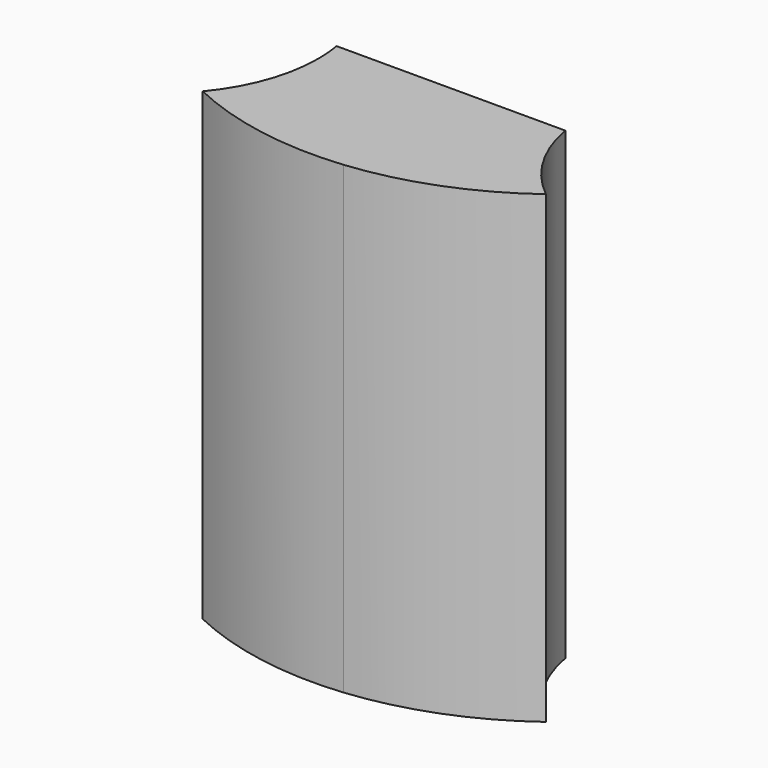
from build123d import *

# Parameters (mm, degrees)
F1_DEPTH = 76.2


with BuildPart() as f1:
    # F0 (on Top) → F1 (new body)
    with BuildSketch(Plane.XY):
        with BuildLine():
            ThreePointArc((5.0166433221, -50.5516892871), (18.3621332827, -47.3653044043), (30.3681236725, -40.7236671312))
            ThreePointArc((30.3681236725, -40.7236671312), (24.4383893444, -33.8843769742), (21.2835539426, -25.4))
            Line((21.2835539426, -25.4), (-16.2238025261, -25.4))
            ThreePointArc((-16.2238025261, -25.4), (-15.9591486415, -27.5028208782), (-15.8707254658, -29.6203852022))
            ThreePointArc((-15.8707254658, -29.6203852022), (-17.3915692894, -38.277515229), (-21.771977458, -45.8979411038))
            ThreePointArc((-21.771977458, -45.8979411038), (-8.6948058368, -50.050378135), (5.0166433221, -50.5516892871))
        make_face()
    extrude(amount=F1_DEPTH)


solid = f1.part
